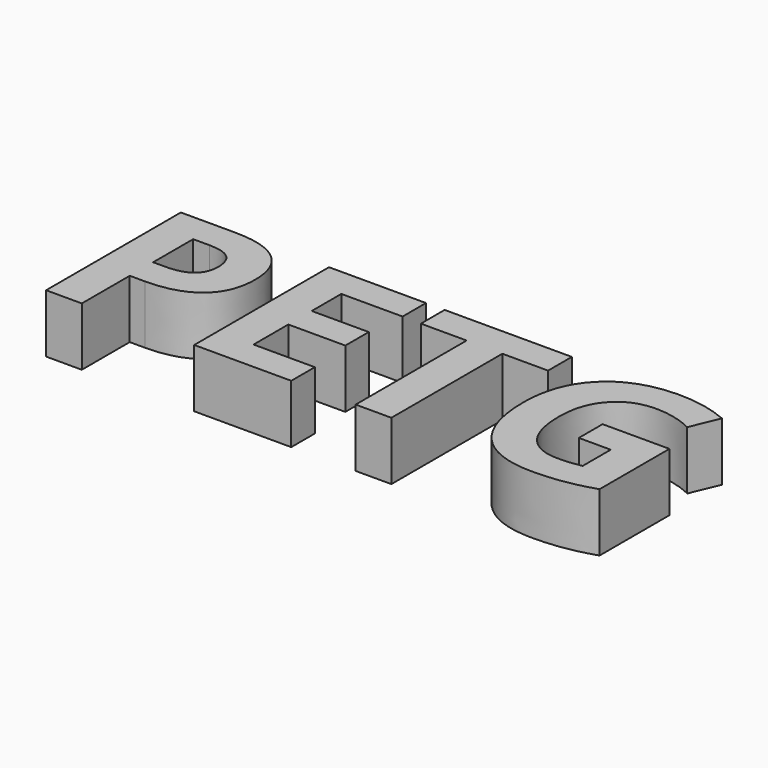
from build123d import *

# Parameters (mm, degrees)
F0_TEXT_SIZE = 40.3887416383
F1_DEPTH     = 10


# Not quite as in the source:
# - Text() gives the source's letters only with a copy of the font that has no kerning and outlines rounded to 1/6400 em; it was checked with that copy


with BuildPart() as f1:
    # F0 (on Top) → F1 (new body)
    with BuildSketch(Plane.XY):
        with Locations((-50, -14.54)):
            Text('PETG', F0_TEXT_SIZE, font='Open Sans', font_style=FontStyle.BOLD, text_align=(TextAlign.LEFT, TextAlign.BOTTOM))
    extrude(amount=F1_DEPTH)


solid = f1.part
